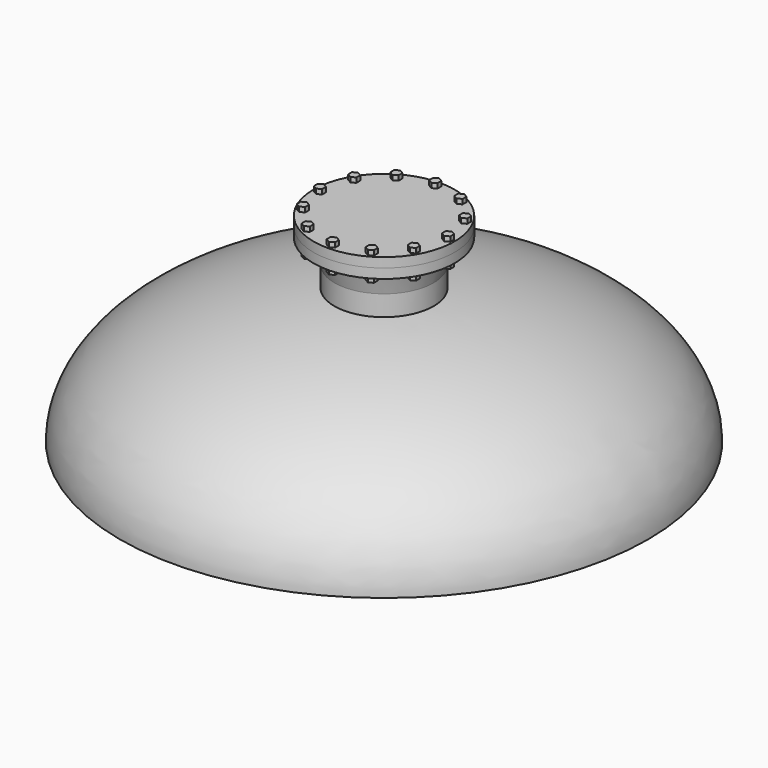
from build123d import *

# Parameters (mm, degrees)
F6_DEPTH  = 1.27
F7_START  = -5.08
F7_DEPTH  = 1.27
F9_R      = 10.5833333333
F10_DEPTH = 254


with BuildPart() as f1:
    # F0 (on Front) → F1 (revolve)
    with BuildSketch(Plane.XZ):
        with BuildLine():
            Line((0, 36.5125), (0, 33.3375))
            add(Edge.make_bspline(
                [(66.675, 0), (66.675, 33.3375), (0, 33.3375)],
                knots=[0, 0, 0, 1.5707963268, 1.5707963268, 1.5707963268], degree=2, weights=[1, 0.7071067812, 1]))
            Line((66.675, 0), (69.85, 0))
            add(Edge.make_bspline(
                [(69.85, 0), (69.85, 36.5125), (0, 36.5125)],
                knots=[0, 0, 0, 1.5707963268, 1.5707963268, 1.5707963268], degree=2, weights=[1, 0.7071067812, 1]))
        make_face()
    revolve(axis=Axis((0, 0, 16.66875), (0, 0, 1)))

    # F9 (on Top) → F10 (cut)
    with BuildSketch(Plane.XY):
        Circle(F9_R)
    extrude(amount=F10_DEPTH, mode=Mode.SUBTRACT)


with BuildPart() as f3:
    # F2 (on Front) → F3 (revolve)
    with BuildSketch(Plane.XZ):
        Polygon((-10.5833333333, 33.02), (-10.5833333333, 34.925), (-10.5833333333, 41.275), (-13.1233333333, 41.275), (-13.1233333333, 33.02), align=None)
        Polygon((-13.1233333333, 41.275), (-10.5833333333, 41.275), (-12.2848107053, 47.625), (-14.8248107053, 47.625), align=None)
        Polygon((-14.8248107053, 47.625), (-12.2848107053, 47.625), (-12.2848107053, 50.165), (-18.6348107053, 50.165), (-18.6348107053, 47.625), align=None)
    revolve(axis=Axis((0, 0, 46.129184404), (0, 0, 1)))

    # F5 (on face) → F7 (join)
    with BuildSketch(Plane.XY.offset(52.705).offset(F7_START)):
        Polygon((1.0998522628, 16.2983333333), (1.0998522628, 17.5683333333), (0, 18.2033333333), (-1.0998522628, 17.5683333333), (-1.0998522628, 16.2983333333), (0, 15.6633333333), align=None)
        Polygon((9.5665189295, 14.0296968374), (9.5665189295, 15.2996968374), (8.4666666667, 15.9346968374), (7.3668144039, 15.2996968374), (7.3668144039, 14.0296968374), (8.4666666667, 13.3946968374), align=None)
        Polygon((15.7645491002, 7.8316666667), (15.7645491002, 9.1016666667), (14.6646968374, 9.7366666667), (13.5648445746, 9.1016666667), (13.5648445746, 7.8316666667), (14.6646968374, 7.1966666667), align=None)
        Polygon((18.0331855961, -0.635), (18.0331855961, 0.635), (16.9333333333, 1.27), (15.8334810705, 0.635), (15.8334810705, -0.635), (16.9333333333, -1.27), align=None)
        Polygon((15.7645491002, -9.1016666667), (15.7645491002, -7.8316666667), (14.6646968374, -7.1966666667), (13.5648445746, -7.8316666667), (13.5648445746, -9.1016666667), (14.6646968374, -9.7366666667), align=None)
        Polygon((9.5665189295, -15.2996968374), (9.5665189295, -14.0296968374), (8.4666666667, -13.3946968374), (7.3668144039, -14.0296968374), (7.3668144039, -15.2996968374), (8.4666666667, -15.9346968374), align=None)
        Polygon((1.0998522628, -17.5683333333), (1.0998522628, -16.2983333333), (0, -15.6633333333), (-1.0998522628, -16.2983333333), (-1.0998522628, -17.5683333333), (0, -18.2033333333), align=None)
        Polygon((-7.3668144039, -15.2996968374), (-7.3668144039, -14.0296968374), (-8.4666666667, -13.3946968374), (-9.5665189295, -14.0296968374), (-9.5665189295, -15.2996968374), (-8.4666666667, -15.9346968374), align=None)
        Polygon((-13.5648445746, -9.1016666667), (-13.5648445746, -7.8316666667), (-14.6646968374, -7.1966666667), (-15.7645491002, -7.8316666667), (-15.7645491002, -9.1016666667), (-14.6646968374, -9.7366666667), align=None)
        Polygon((-15.8334810705, -0.635), (-15.8334810705, 0.635), (-16.9333333333, 1.27), (-18.0331855961, 0.635), (-18.0331855961, -0.635), (-16.9333333333, -1.27), align=None)
        Polygon((-13.5648445746, 7.8316666667), (-13.5648445746, 9.1016666667), (-14.6646968374, 9.7366666667), (-15.7645491002, 9.1016666667), (-15.7645491002, 7.8316666667), (-14.6646968374, 7.1966666667), align=None)
        Polygon((-7.3668144039, 14.0296968374), (-7.3668144039, 15.2996968374), (-8.4666666667, 15.9346968374), (-9.5665189295, 15.2996968374), (-9.5665189295, 14.0296968374), (-8.4666666667, 13.3946968374), align=None)
    extrude(amount=-F7_DEPTH)

    # F0 (on Front) → F8 (revolve, cut)
    with BuildSketch(Plane.XZ):
        with BuildLine():
            Line((0, 36.5125), (0, 33.3375))
            add(Edge.make_bspline(
                [(66.675, 0), (66.675, 33.3375), (0, 33.3375)],
                knots=[0, 0, 0, 1.5707963268, 1.5707963268, 1.5707963268], degree=2, weights=[1, 0.7071067812, 1]))
            Line((66.675, 0), (69.85, 0))
            add(Edge.make_bspline(
                [(69.85, 0), (69.85, 36.5125), (0, 36.5125)],
                knots=[0, 0, 0, 1.5707963268, 1.5707963268, 1.5707963268], degree=2, weights=[1, 0.7071067812, 1]))
        make_face()
    revolve(axis=Axis((0, 0, 16.66875), (0, 0, 1)), mode=Mode.SUBTRACT)


with BuildPart() as f4:
    # F2 (on Front) → F4 (revolve)
    with BuildSketch(Plane.XZ):
        Polygon((-18.6348107053, 50.165), (-12.2848107053, 50.165), (0, 50.165), (0, 52.705), (-18.6348107053, 52.705), align=None)
    revolve(axis=Axis((0, 0, 46.129184404), (0, 0, 1)))

    # F5 (on face) → F6 (join)
    with BuildSketch(Plane.XY.offset(52.705)):
        Polygon((1.0998522628, 16.2983333333), (1.0998522628, 17.5683333333), (0, 18.2033333333), (-1.0998522628, 17.5683333333), (-1.0998522628, 16.2983333333), (0, 15.6633333333), align=None)
        Polygon((9.5665189295, 14.0296968374), (9.5665189295, 15.2996968374), (8.4666666667, 15.9346968374), (7.3668144039, 15.2996968374), (7.3668144039, 14.0296968374), (8.4666666667, 13.3946968374), align=None)
        Polygon((15.7645491002, 7.8316666667), (15.7645491002, 9.1016666667), (14.6646968374, 9.7366666667), (13.5648445746, 9.1016666667), (13.5648445746, 7.8316666667), (14.6646968374, 7.1966666667), align=None)
        Polygon((18.0331855961, -0.635), (18.0331855961, 0.635), (16.9333333333, 1.27), (15.8334810705, 0.635), (15.8334810705, -0.635), (16.9333333333, -1.27), align=None)
        Polygon((15.7645491002, -9.1016666667), (15.7645491002, -7.8316666667), (14.6646968374, -7.1966666667), (13.5648445746, -7.8316666667), (13.5648445746, -9.1016666667), (14.6646968374, -9.7366666667), align=None)
        Polygon((9.5665189295, -15.2996968374), (9.5665189295, -14.0296968374), (8.4666666667, -13.3946968374), (7.3668144039, -14.0296968374), (7.3668144039, -15.2996968374), (8.4666666667, -15.9346968374), align=None)
        Polygon((1.0998522628, -17.5683333333), (1.0998522628, -16.2983333333), (0, -15.6633333333), (-1.0998522628, -16.2983333333), (-1.0998522628, -17.5683333333), (0, -18.2033333333), align=None)
        Polygon((-7.3668144039, -15.2996968374), (-7.3668144039, -14.0296968374), (-8.4666666667, -13.3946968374), (-9.5665189295, -14.0296968374), (-9.5665189295, -15.2996968374), (-8.4666666667, -15.9346968374), align=None)
        Polygon((-13.5648445746, -9.1016666667), (-13.5648445746, -7.8316666667), (-14.6646968374, -7.1966666667), (-15.7645491002, -7.8316666667), (-15.7645491002, -9.1016666667), (-14.6646968374, -9.7366666667), align=None)
        Polygon((-15.8334810705, -0.635), (-15.8334810705, 0.635), (-16.9333333333, 1.27), (-18.0331855961, 0.635), (-18.0331855961, -0.635), (-16.9333333333, -1.27), align=None)
        Polygon((-13.5648445746, 7.8316666667), (-13.5648445746, 9.1016666667), (-14.6646968374, 9.7366666667), (-15.7645491002, 9.1016666667), (-15.7645491002, 7.8316666667), (-14.6646968374, 7.1966666667), align=None)
        Polygon((-7.3668144039, 14.0296968374), (-7.3668144039, 15.2996968374), (-8.4666666667, 15.9346968374), (-9.5665189295, 15.2996968374), (-9.5665189295, 14.0296968374), (-8.4666666667, 13.3946968374), align=None)
    extrude(amount=F6_DEPTH)


solid = Compound([f1.part, f3.part, f4.part])
